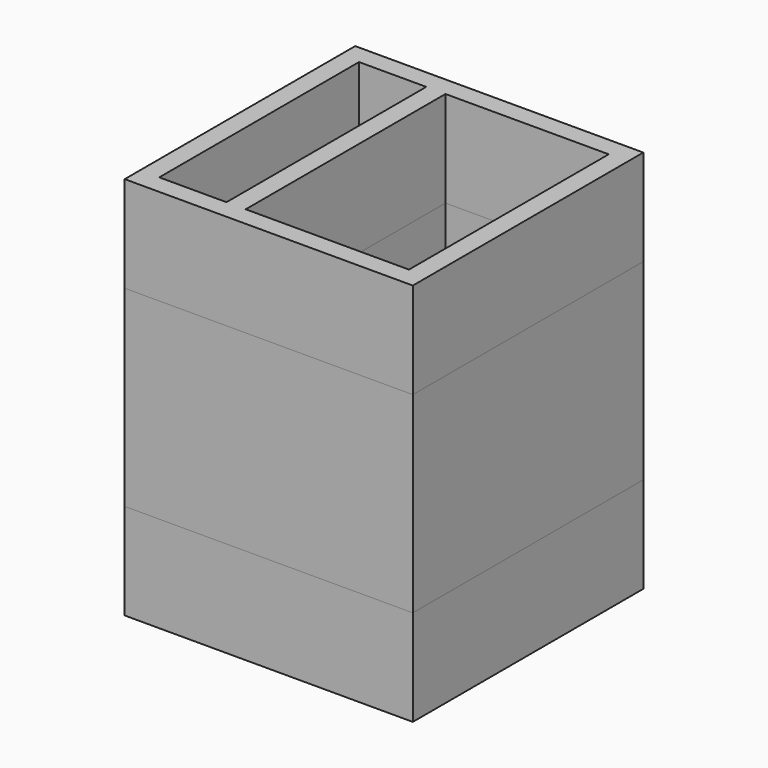
from build123d import *

# Parameters (mm, degrees)
F0_W        = 76.2
F0_H        = 76.2
F0_W_2      = 5.08
F0_H_2      = 66.04
F1_DEPTH    = 76.2
F0_W_3      = 43.18
F1_FACE_W   = 76.2
F1_FACE_H   = 76.2
F1_FACE_W_2 = 43.18
F1_FACE_H_2 = 66.04
F1_FACE_W_3 = 17.78
F2_DEPTH    = 25.4


# Not quite as in the source:
# - a feature names something its author has since deleted; it is built from what else it names


with BuildPart() as f1:
    # F0 (on Top) → F1 (new body)
    with BuildSketch(Plane.XY):
        Rectangle(F0_W, F0_H)
        Polygon((-10.16, 33.02), (33.02, 33.02), (33.02, -33.02), (-10.16, -33.02), (-15.24, -33.02), (-33.02, -33.02), (-33.02, 33.02), (-15.24, 33.02), align=None, mode=Mode.SUBTRACT)
        with Locations((-12.7, 0)):
            Rectangle(F0_W_2, F0_H_2)
    extrude(amount=F1_DEPTH)


with BuildPart() as f2:
    # F0 (on Top) + F1_face (on face) → F2 (new body)
    with BuildSketch(Plane.XY):
        Rectangle(F0_W, F0_H)
        Polygon((-10.16, 33.02), (33.02, 33.02), (33.02, -33.02), (-10.16, -33.02), (-15.24, -33.02), (-33.02, -33.02), (-33.02, 33.02), (-15.24, 33.02), align=None, mode=Mode.SUBTRACT)
        with Locations((11.43, 0)):
            Rectangle(F0_W_3, F0_H_2)
    with BuildSketch(Plane(origin=(-2.3927536232, 0, 76.2), x_dir=(1, 0, 0), z_dir=(0, 0, 1))):
        with Locations((2.3927536232, 0)):
            Rectangle(F1_FACE_W, F1_FACE_H)
        with Locations((13.8227536232, 0)):
            Rectangle(F1_FACE_W_2, F1_FACE_H_2, mode=Mode.SUBTRACT)
        with Locations((-21.7372463768, 0)):
            Rectangle(F1_FACE_W_3, F1_FACE_H_2, mode=Mode.SUBTRACT)
    extrude(amount=F2_DEPTH)


solid = Compound([f1.part, f2.part])
